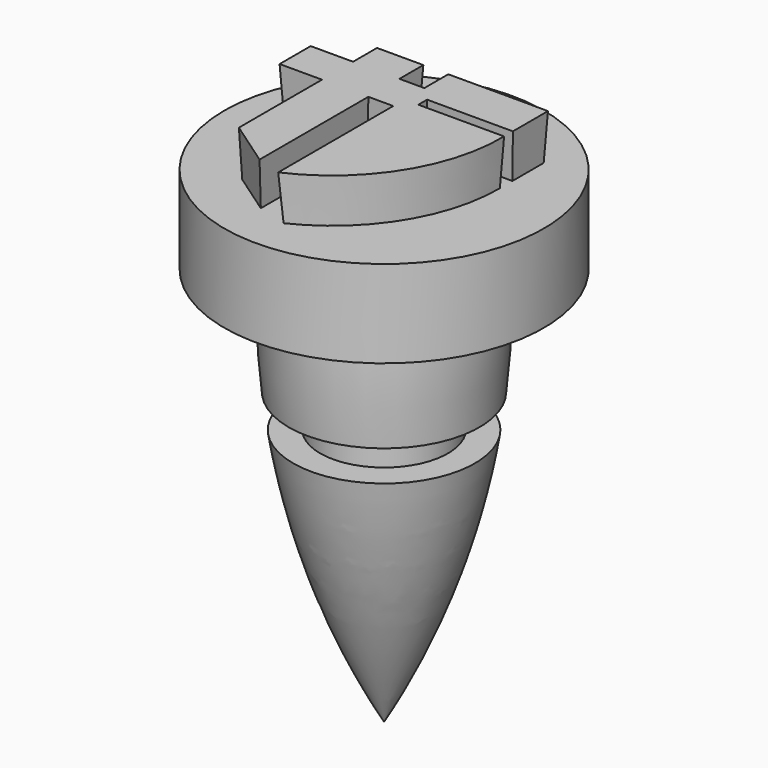
from build123d import *

# Parameters (mm, degrees)
F3_DEPTH                 = 12.7
DRAFT_F3_DRAFTED_ANGLE   = -3
DRAFT_F3_2_DRAFTED_ANGLE = -3
F2_W                     = 8.1924527405
F2_H                     = 2.8575000616
DRAFT_F3_3_DRAFTED_ANGLE = -3


# Not quite as in the source:
# - an extrude with a draft is written as a straight extrude whose walls are then drafted


with BuildPart() as f1:
    # F0 (on Front) → F1 (revolve)
    with BuildSketch(Plane.XZ):
        with BuildLine():
            Line((0, -38.1), (0, 0))
            Line((0, 0), (0, 8.3553222939))
            Line((0, 8.3553222939), (-15.2647523209, 8.3553222939))
            Line((-15.2647523209, 8.3553222939), (-15.2647523209, 0))
            Line((-15.2647523209, 0), (-9.525, 0))
            ThreePointArc((-9.525, 0), (-9.5066691574, -5.1848451048), (-9.1134021831, -10.3547866778))
            Line((-9.1134021831, -10.3547866778), (-6.1057287889, -10.3547866778))
            Line((-6.1057287889, -10.3547866778), (-6.1057287889, -13.5297866778))
            Line((-6.1057287889, -13.5297866778), (-8.6838452705, -13.5297866778))
            ThreePointArc((-8.6838452705, -13.5297866778), (-5.4684636958, -26.2130465064), (0, -38.1))
        make_face()
    revolve(axis=Axis((0, 0, -19.05), (0, 0, -1)))


with BuildPart() as f3_drafted:
    # F2 (on Top) → F3 (new body)
    with BuildSketch(Plane.XY):
        Polygon((-3.7137963349, 2.5931939593), (0, 2.5931939593), (0, 4.9744433429), (-3.7137963349, 4.9744433429), (-3.7137963349, 7.8319434046), (-6.8094214274, 7.8319434046), (-6.8094214274, 4.9744433429), (-10.8575472595, 4.9744433429), (-10.8575472595, 2.5931939593), (-6.8094214274, 2.5931939593), (-6.8094214274, -7.6461802086), (-3.7137963349, -9.7893045614), align=None)
    extrude(amount=F3_DEPTH)

    # draft_F3_drafted
    draft_f3_drafted_walls = [f3_drafted.faces().sort_by_distance(p)[0] for p in [
        (-6.8094214274, -2.5264931246, 8.4666666667),
        (-5.2616088812, -8.717742385, 8.4666666667),
        (-3.7137963349, -3.598055301, 8.4666666667),
        (-1.8568981675, 2.5931939593, 8.4666666667),
        (0, 3.7838186511, 8.4666666667),
        (-1.8568981675, 4.9744433429, 8.4666666667),
        (-3.7137963349, 6.4031933738, 8.4666666667),
        (-5.2616088812, 7.8319434046, 8.4666666667),
        (-6.8094214274, 6.4031933738, 8.4666666667),
        (-8.8334843434, 4.9744433429, 8.4666666667),
        (-10.8575472595, 3.7838186511, 8.4666666667),
        (-8.8334843434, 2.5931939593, 8.4666666667),
    ]]
    draft(draft_f3_drafted_walls, neutral_plane=Plane.XY, angle=DRAFT_F3_DRAFTED_ANGLE)


with BuildPart() as f1_1:
    add(f1.part)

    # join_F3_drafted: union F3_drafted
    add(f3_drafted.part)


with BuildPart() as f3_2_drafted:
    # F2 (on Top) → F3, piece 2 (new body)
    with BuildSketch(Plane.XY):
        with BuildLine():
            Line((8.1924527405, 2.5931939593), (0, 2.5931939593))
            Line((0, 2.5931939593), (0, -10.7418046847))
            ThreePointArc((0, -10.7418046847), (5.8999730413, -5.1824501592), (8.1924527405, 2.5931939593))
        make_face()
    extrude(amount=F3_DEPTH)

    # draft_F3_2_drafted
    draft_f3_2_drafted_walls = [f3_2_drafted.faces().sort_by_distance(p)[0] for p in [
        (4.0962263703, 2.5931939593, 8.4666666667),
        (0, -4.0743053627, 8.4666666667),
        (5.8999730413, -5.1824501592, 8.4666666667),
    ]]
    draft(draft_f3_2_drafted_walls, neutral_plane=Plane.XY, angle=DRAFT_F3_2_DRAFTED_ANGLE)


with BuildPart() as f1_2:
    add(f1_1.part)

    # join_F3_2_drafted: union F3_2_drafted
    add(f3_2_drafted.part)


with BuildPart() as f3_3_drafted:
    # F2 (on Top) → F3, piece 3 (new body)
    with BuildSketch(Plane.XY):
        with Locations((4.0962263703, 6.4031933738)):
            Rectangle(F2_W, F2_H)
    extrude(amount=F3_DEPTH)

    # draft_F3_3_drafted
    draft_f3_3_drafted_walls = [f3_3_drafted.faces().sort_by_distance(p)[0] for p in [
        (8.1924527405, 6.4031933738, 8.4666666667),
        (4.0962263703, 7.8319434046, 8.4666666667),
        (0, 6.4031933738, 8.4666666667),
        (4.0962263703, 4.9744433429, 8.4666666667),
    ]]
    draft(draft_f3_3_drafted_walls, neutral_plane=Plane.XY, angle=DRAFT_F3_3_DRAFTED_ANGLE)


with BuildPart() as f1_3:
    add(f1_2.part)

    # join_F3_3_drafted: union F3_3_drafted
    add(f3_3_drafted.part)


solid = f1_3.part
